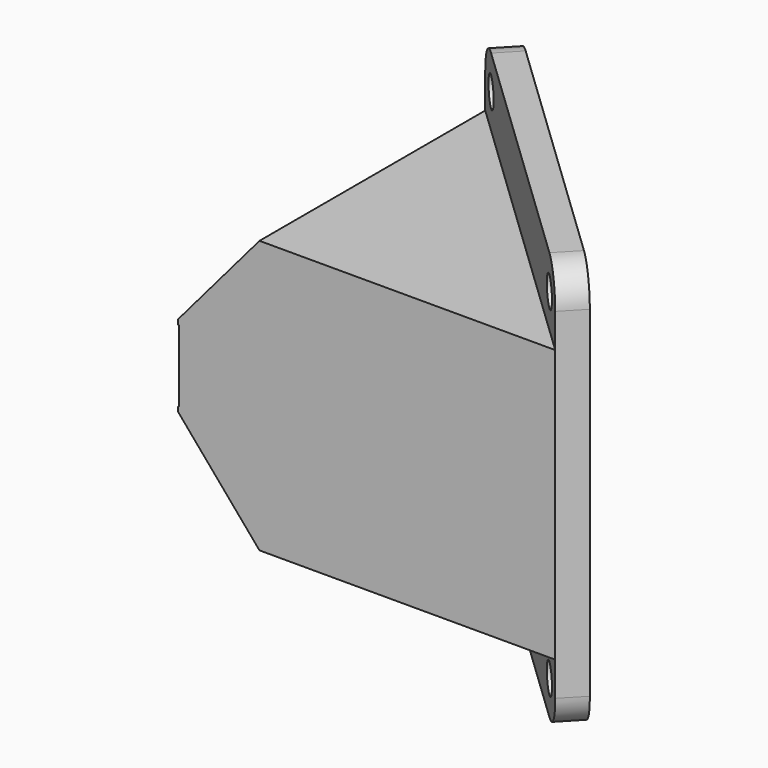
from build123d import *

# Parameters (mm, degrees)
F1_DEPTH = 31.75
F3_REACH = 47.4787425117
F4_T     = -1.5875
F5_W     = 3.0979418965
F5_H     = 8.3555914986
F6_REACH = 39.2365913389
F7_W     = 47.625
F7_H     = 7.9375
F7_R     = 1.7272
F7_H_2   = 31.75
F7_W_2   = 43.5875253129
F7_H_3   = 28.575
F8_DEPTH = 3.175
F9_R     = 3.96875


with BuildPart() as f1:
    # F0 (on Top) → F1 (new body)
    with BuildSketch(Plane.XY):
        Polygon((-43.9269818101, 0), (0, 0), (-34.4563574527, 32.8770445158), (-43.9269818101, 6.35), align=None)
    extrude(amount=F1_DEPTH)

    f3_end = f1.faces().sort_by_distance((-39.1916696314, 19.6135222579, 15.875))[0]
    # F2 (on face) → F3 (cut, up to a face of the model that its end follows)
    with BuildSketch(Plane.XZ):
        Polygon((-43.9269818101, 11.1125), (-43.9269818101, 0), (-34.4563574527, 0), align=None)
        Polygon((-34.4563574527, 31.75), (-43.9269818101, 31.75), (-43.9269818101, 20.6375), align=None)
    f3_long = extrude(amount=-F3_REACH, mode=Mode.PRIVATE)
    add(split(f3_long, bisect_by=f3_end, keep=Keep.BOTTOM, mode=Mode.PRIVATE), mode=Mode.SUBTRACT)

    # F4
    f4_openings = [f1.faces().sort_by_distance(p)[0] for p in [
        (-17.228179, 16.438522, 15.875),
    ]]
    offset(amount=F4_T, openings=f4_openings)

    f6_end = Plane(origin=(-43.9269818101, 3.175, 15.875), x_dir=(0, 0, -1), z_dir=(-1, 0, 0))
    # F5 (on face) → F6 (cut, up to a plane its end follows)
    with BuildSketch(Plane(origin=(0, 0, 0), x_dir=(-0.7234930699, 0.6903316434, 0), z_dir=(0.6903316434, 0.7234930699, 0))):
        with Locations((33.2771941037, 15.875)):
            Rectangle(F5_W, F5_H)
    f6_long = extrude(amount=-F6_REACH, mode=Mode.PRIVATE)
    add(split(f6_long, bisect_by=f6_end, keep=Keep.BOTTOM, mode=Mode.PRIVATE), mode=Mode.SUBTRACT)

    # F7 (on face) → F8 (join)
    with BuildSketch(Plane(origin=(0, 0, 0), x_dir=(-0.7234930699, 0.6903316434, 0), z_dir=(0.6903316434, 0.7234930699, 0))):
        with Locations((23.8125, -3.96875)):
            Rectangle(F7_W, F7_H)
        with Locations((3.96875, -3.96875)):
            Circle(F7_R, mode=Mode.SUBTRACT)
        with Locations((43.65625, -3.96875)):
            Circle(F7_R, mode=Mode.SUBTRACT)
        with Locations((23.8125, 35.71875)):
            Rectangle(F7_W, F7_H)
        with Locations((3.96875, 35.71875)):
            Circle(F7_R, mode=Mode.SUBTRACT)
        with Locations((43.65625, 35.71875)):
            Circle(F7_R, mode=Mode.SUBTRACT)
        with Locations((23.8125, 15.875)):
            Rectangle(F7_W, F7_H_2)
        with Locations((24.0933819992, 15.875)):
            Rectangle(F7_W_2, F7_H_3, mode=Mode.SUBTRACT)
    extrude(amount=F8_DEPTH)

    # F9
    f9_edges = [f1.edges().sort_by_distance(p)[0] for p in [
        (-33.360456, 34.02559, -7.9375),
        (1.095901, 1.148545, -7.9375),
        (-33.360456, 34.02559, 39.6875),
        (1.095901, 1.148545, 39.6875),
    ]]
    fillet(f9_edges, radius=F9_R)


solid = f1.part
